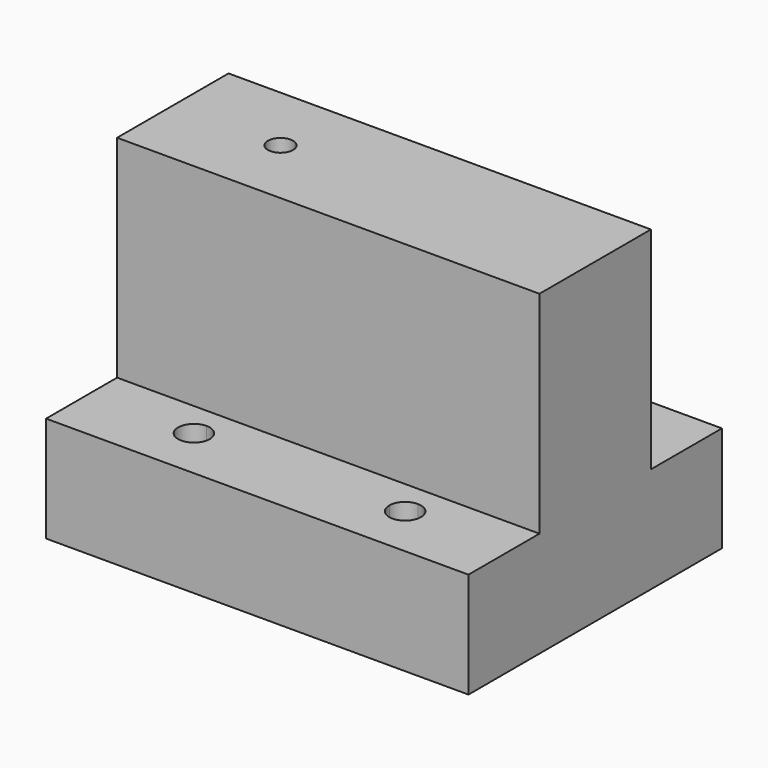
from build123d import *

# Parameters (mm, degrees)
F0_W     = 101.6
F0_H     = 76.2
F1_DEPTH = 25.4
F2_W     = 101.6
F2_H     = 33.5062108934
F3_DEPTH = 50.8
F4_R     = 1.0287
F5_DEPTH = 101.6
F6_R     = 3.0226
F6_R_2   = 1.0287
F7_DEPTH = 38.1


with BuildPart() as f1:
    # F0 (on Top) → F1 (new body)
    with BuildSketch(Plane.XY):
        Rectangle(F0_W, F0_H)
        with BuildLine():
            ThreePointArc((-25.4, 21.59), (-28.0940768363, 28.0940768363), (-21.59, 25.4))
            Line((-21.59, 25.4), (21.59, 25.4))
            ThreePointArc((21.59, 25.4), (25.4, 29.21), (29.21, 25.4))
            ThreePointArc((29.21, 25.4), (28.0940768363, 22.7059231637), (25.4, 21.59))
            Line((25.4, 21.59), (25.4, -21.59))
            ThreePointArc((25.4, -21.59), (28.0940768363, -22.7059231637), (29.21, -25.4))
            ThreePointArc((29.21, -25.4), (25.4, -29.21), (21.59, -25.4))
            Line((21.59, -25.4), (-21.59, -25.4))
            ThreePointArc((-21.59, -25.4), (-28.0940768363, -28.0940768363), (-25.4, -21.59))
            Line((-25.4, -21.59), (-25.4, 21.59))
        make_face(mode=Mode.SUBTRACT)
        with BuildLine():
            Line((21.59, 25.4), (-21.59, 25.4))
            ThreePointArc((-21.59, 25.4), (-22.7059231637, 22.7059231637), (-25.4, 21.59))
            Line((-25.4, 21.59), (-25.4, -21.59))
            ThreePointArc((-25.4, -21.59), (-22.7059231637, -22.7059231637), (-21.59, -25.4))
            Line((-21.59, -25.4), (21.59, -25.4))
            ThreePointArc((21.59, -25.4), (22.7059231637, -22.7059231637), (25.4, -21.59))
            Line((25.4, -21.59), (25.4, 21.59))
            ThreePointArc((25.4, 21.59), (22.7059231637, 22.7059231637), (21.59, 25.4))
        make_face()
    extrude(amount=F1_DEPTH)

    # F2 (on face) → F3 (join)
    with BuildSketch(Plane.XY.offset(25.4)):
        Rectangle(F2_W, F2_H)
    extrude(amount=F3_DEPTH)

    # F4 (on face) → F5 (cut)
    with BuildSketch(Plane.XY.offset(76.2)):
        with Locations((-24.892, 0)):
            Circle(F4_R)
    extrude(amount=-F5_DEPTH, mode=Mode.SUBTRACT)

    # F6 (on face) → F7 (cut)
    with BuildSketch(Plane.XY.offset(76.2)):
        with Locations((-24.892, 0)):
            Circle(F6_R)
        with Locations((-24.892, 0)):
            Circle(F6_R_2, mode=Mode.SUBTRACT)
    extrude(amount=-F7_DEPTH, mode=Mode.SUBTRACT)


solid = f1.part
